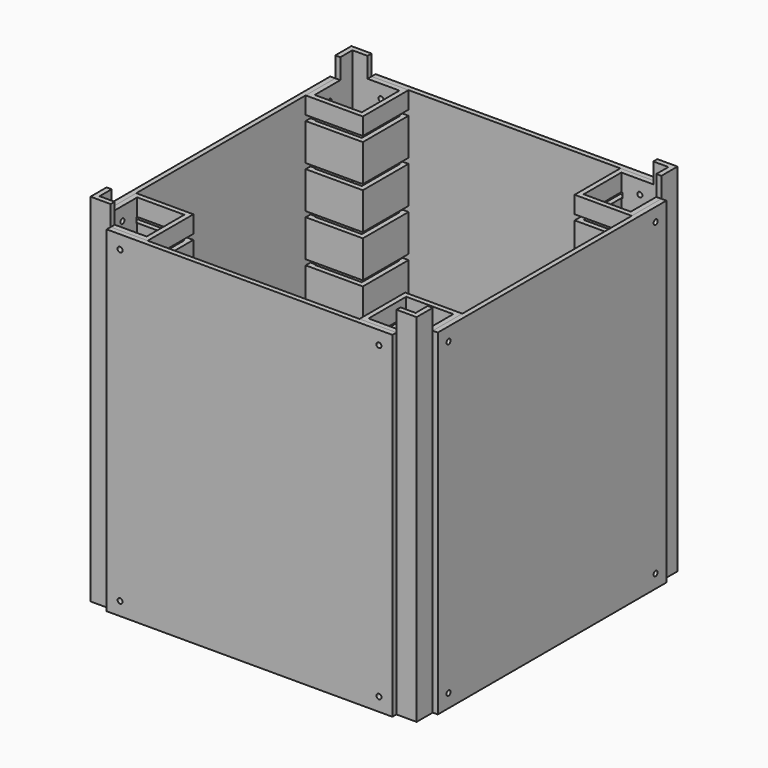
from build123d import *

# Parameters (mm, degrees)
F0_W      = 14
F0_H      = 14
F1_DEPTH  = 100
F2_W      = 85
F2_H      = 1.5
F3_DEPTH  = 100
F2_W_2    = 1.5
F2_H_2    = 85
F5_DEPTH  = 6
F6_R      = 0.75
F7_DEPTH  = 10
F8_R      = 0.75
F9_DEPTH  = 10
F10_R     = 0.75
F11_DEPTH = 10
F12_R     = 0.75
F13_DEPTH = 10
F14_W     = 17
F14_H     = 1.6
F15_DEPTH = 1.8
F16_W     = 17
F16_H     = 1.6
F17_DEPTH = 1.8
F18_W     = 17
F18_H     = 1.6
F19_DEPTH = 1.8
F20_W     = 17
F20_H     = 1.6
F21_DEPTH = 1.8
F22_W     = 17
F22_H     = 1.6
F23_DEPTH = 1.8
F24_W     = 17
F24_H     = 1.6
F25_DEPTH = 1.8
F26_W     = 17
F26_H     = 1.6
F27_DEPTH = 1.8
F28_W     = 17
F28_H     = 1.6
F29_DEPTH = 1.8
F30_W     = 17
F30_H     = 1.6
F31_DEPTH = 1.8
F32_W     = 17
F32_H     = 1.6
F33_DEPTH = 1.8


with BuildPart() as f1:
    # F0 (on Top) → F1 (new body)
    with BuildSketch(Plane.XY):
        Polygon((17, 97), (0, 97), (0, 95.5), (0, 80), (1.5, 80), (15.5, 80), (17, 80), (17, 95.5), align=None)
        with Locations((8.5, 88.5)):
            Rectangle(F0_W, F0_H, mode=Mode.SUBTRACT)
    extrude(amount=-F1_DEPTH)

    # F4 (on face) → F5 (join)
    with BuildSketch(Plane.XY):
        Polygon((6, 97), (0, 97), (0, 91), (1.5, 91), (1.5, 95.5), (6, 95.5), align=None)
    extrude(amount=F5_DEPTH)


with BuildPart() as f1b:
    # F0 (on Top) → F1, piece 2 (new body)
    with BuildSketch(Plane.XY):
        Polygon((97, 97), (80, 97), (80, 95.5), (80, 80), (81.5, 80), (95.5, 80), (97, 80), (97, 95.5), align=None)
        with Locations((88.5, 88.5)):
            Rectangle(F0_W, F0_H, mode=Mode.SUBTRACT)
    extrude(amount=-F1_DEPTH)

    # F4 (on face) → F5, piece 2 (join)
    with BuildSketch(Plane.XY):
        Polygon((97, 97), (91, 97), (91, 95.5), (95.5, 95.5), (95.5, 91), (97, 91), align=None)
    extrude(amount=F5_DEPTH)


with BuildPart() as f1c:
    # F0 (on Top) → F1, piece 3 (new body)
    with BuildSketch(Plane.XY):
        Polygon((95.5, 0), (97, 0), (97, 15.5), (97, 17), (80, 17), (80, 15.5), (80, 0), (81.5, 0), align=None)
        with Locations((88.5, 8.5)):
            Rectangle(F0_W, F0_H, mode=Mode.SUBTRACT)
    extrude(amount=-F1_DEPTH)

    # F4 (on face) → F5, piece 3 (join)
    with BuildSketch(Plane.XY):
        Polygon((97, 0), (97, 6), (95.5, 6), (95.5, 1.5), (91, 1.5), (91, 0), align=None)
    extrude(amount=F5_DEPTH)


with BuildPart() as f1d:
    # F0 (on Top) → F1, piece 4 (new body)
    with BuildSketch(Plane.XY):
        Polygon((17, 15.5), (17, 17), (0, 17), (0, 15.5), (0, 0), (1.5, 0), (15.5, 0), (17, 0), align=None)
        with Locations((8.5, 8.5)):
            Rectangle(F0_W, F0_H, mode=Mode.SUBTRACT)
    extrude(amount=-F1_DEPTH)

    # F4 (on face) → F5, piece 4 (join)
    with BuildSketch(Plane.XY):
        Polygon((1.5, 6), (0, 6), (0, 0), (6, 0), (6, 1.5), (1.5, 1.5), align=None)
    extrude(amount=F5_DEPTH)


with BuildPart() as f3:
    # F2 (on face) → F3 (new body)
    with BuildSketch(Plane.XY):
        with Locations((48.5, -0.75)):
            Rectangle(F2_W, F2_H)
    extrude(amount=-F3_DEPTH)


with BuildPart() as f3b:
    # F2 (on face) → F3, piece 2 (new body)
    with BuildSketch(Plane.XY):
        with Locations((-0.75, 48.5)):
            Rectangle(F2_W_2, F2_H_2)
    extrude(amount=-F3_DEPTH)


with BuildPart() as f3c:
    # F2 (on face) → F3, piece 3 (new body)
    with BuildSketch(Plane.XY):
        Polygon((98.5, 91), (97, 91), (97, 80), (97, 17), (97, 6), (98.5, 6), align=None)
    extrude(amount=-F3_DEPTH)


with BuildPart() as f3d:
    # F2 (on face) → F3, piece 4 (new body)
    with BuildSketch(Plane.XY):
        Polygon((6, 98.5), (6, 97), (80, 97), (91, 97), (91, 98.5), align=None)
    extrude(amount=-F3_DEPTH)


with BuildPart() as f7_tool:
    # F6 (on face) → F7 (new body)
    with BuildSketch(Plane.YZ.offset(98.5)):
        with Locations((10, -4)):
            Circle(F6_R)
        with Locations((87, -4)):
            Circle(F6_R)
        with Locations((87, -96)):
            Circle(F6_R)
        with Locations((10, -96)):
            Circle(F6_R)
    extrude(amount=-F7_DEPTH)


with BuildPart() as f1b_1:
    add(f1b.part)

    # F7: cut by f7_tool
    add(f7_tool.part, mode=Mode.SUBTRACT)


with BuildPart() as f1c_1:
    add(f1c.part)

    # F7: cut by f7_tool
    add(f7_tool.part, mode=Mode.SUBTRACT)


with BuildPart() as f3c_1:
    add(f3c.part)

    # F7: cut by f7_tool
    add(f7_tool.part, mode=Mode.SUBTRACT)


with BuildPart() as f9_tool:
    # F8 (on face) → F9 (new body)
    with BuildSketch(Plane(origin=(0, 98.5, 0), x_dir=(-1, 0, 0), z_dir=(0, 1, 0))):
        with Locations((-87, -4)):
            Circle(F8_R)
        with Locations((-10, -4)):
            Circle(F8_R)
        with Locations((-10, -96)):
            Circle(F8_R)
        with Locations((-87, -96)):
            Circle(F8_R)
    extrude(amount=-F9_DEPTH)


with BuildPart() as f1_1:
    add(f1.part)

    # F9: cut by f9_tool
    add(f9_tool.part, mode=Mode.SUBTRACT)


with BuildPart() as f1b_2:
    add(f1b_1.part)

    # F9: cut by f9_tool
    add(f9_tool.part, mode=Mode.SUBTRACT)

    # F22 (on face) → F23 (cut)
    with BuildSketch(Plane.XZ.offset(-80)):
        with Locations((88.5, -5.91)):
            Rectangle(F22_W, F22_H)
        with Locations((88.5, -18.51)):
            Rectangle(F22_W, F22_H)
        with Locations((88.5, -31.11)):
            Rectangle(F22_W, F22_H)
        with Locations((88.5, -43.71)):
            Rectangle(F22_W, F22_H)
        with Locations((88.5, -56.31)):
            Rectangle(F22_W, F22_H)
        with Locations((88.5, -68.91)):
            Rectangle(F22_W, F22_H)
        with Locations((88.5, -81.51)):
            Rectangle(F22_W, F22_H)
        with Locations((88.5, -94.11)):
            Rectangle(F22_W, F22_H)
    extrude(amount=-F23_DEPTH, mode=Mode.SUBTRACT)

    # F24 (on face) → F25 (cut)
    with BuildSketch(Plane(origin=(80, 0, 0), x_dir=(0, -1, 0), z_dir=(-1, 0, 0))):
        with Locations((-88.5, -5.91)):
            Rectangle(F24_W, F24_H)
        with Locations((-88.5, -18.51)):
            Rectangle(F24_W, F24_H)
        with Locations((-88.5, -31.11)):
            Rectangle(F24_W, F24_H)
        with Locations((-88.5, -43.71)):
            Rectangle(F24_W, F24_H)
        with Locations((-88.5, -56.31)):
            Rectangle(F24_W, F24_H)
        with Locations((-88.5, -68.91)):
            Rectangle(F24_W, F24_H)
        with Locations((-88.5, -81.51)):
            Rectangle(F24_W, F24_H)
        with Locations((-88.5, -94.11)):
            Rectangle(F24_W, F24_H)
    extrude(amount=-F25_DEPTH, mode=Mode.SUBTRACT)


with BuildPart() as f3d_1:
    add(f3d.part)

    # F9: cut by f9_tool
    add(f9_tool.part, mode=Mode.SUBTRACT)


with BuildPart() as f11_tool:
    # F10 (on face) → F11 (new body)
    with BuildSketch(Plane(origin=(-1.5, 0, 0), x_dir=(0, -1, 0), z_dir=(-1, 0, 0))):
        with Locations((-87, -96)):
            Circle(F10_R)
        with Locations((-10, -96)):
            Circle(F10_R)
        with Locations((-10, -4)):
            Circle(F10_R)
        with Locations((-87, -4)):
            Circle(F10_R)
    extrude(amount=-F11_DEPTH)


with BuildPart() as f1_2:
    add(f1_1.part)

    # F11: cut by f11_tool
    add(f11_tool.part, mode=Mode.SUBTRACT)

    # F14 (on face) → F15 (cut)
    with BuildSketch(Plane.XZ.offset(-80)):
        with Locations((8.5, -5.91)):
            Rectangle(F14_W, F14_H)
    extrude(amount=-F15_DEPTH, mode=Mode.SUBTRACT)

    # F16 (on face) → F17 (cut)
    with BuildSketch(Plane.YZ.offset(17)):
        with Locations((88.5, -5.91)):
            Rectangle(F16_W, F16_H)
    extrude(amount=-F17_DEPTH, mode=Mode.SUBTRACT)

    # F18 (on face) → F19 (cut)
    with BuildSketch(Plane.XZ.offset(-80)):
        with Locations((8.5, -94.11)):
            Rectangle(F18_W, F18_H)
        with Locations((8.5, -81.51)):
            Rectangle(F18_W, F18_H)
        with Locations((8.5, -68.91)):
            Rectangle(F18_W, F18_H)
        with Locations((8.5, -56.31)):
            Rectangle(F18_W, F18_H)
        with Locations((8.5, -43.71)):
            Rectangle(F18_W, F18_H)
        with Locations((8.5, -31.11)):
            Rectangle(F18_W, F18_H)
        with Locations((8.5, -18.51)):
            Rectangle(F18_W, F18_H)
    extrude(amount=-F19_DEPTH, mode=Mode.SUBTRACT)

    # F20 (on face) → F21 (cut)
    with BuildSketch(Plane.YZ.offset(17)):
        with Locations((88.5, -18.51)):
            Rectangle(F20_W, F20_H)
        with Locations((88.5, -31.11)):
            Rectangle(F20_W, F20_H)
        with Locations((88.5, -43.71)):
            Rectangle(F20_W, F20_H)
        Polygon((97, -55.51), (81.8, -55.51), (80, -55.51), (80, -57.11), (97, -57.11), align=None)
        with Locations((88.5, -68.91)):
            Rectangle(F20_W, F20_H)
        with Locations((88.5, -81.51)):
            Rectangle(F20_W, F20_H)
        with Locations((88.5, -94.11)):
            Rectangle(F20_W, F20_H)
    extrude(amount=-F21_DEPTH, mode=Mode.SUBTRACT)


with BuildPart() as f1d_1:
    add(f1d.part)

    # F11: cut by f11_tool
    add(f11_tool.part, mode=Mode.SUBTRACT)


with BuildPart() as f3b_1:
    add(f3b.part)

    # F11: cut by f11_tool
    add(f11_tool.part, mode=Mode.SUBTRACT)


with BuildPart() as f13_tool:
    # F12 (on face) → F13 (new body)
    with BuildSketch(Plane.XZ.offset(1.5)):
        with Locations((10, -4)):
            Circle(F12_R)
        with Locations((87, -4)):
            Circle(F12_R)
        with Locations((87, -96)):
            Circle(F12_R)
        with Locations((10, -96)):
            Circle(F12_R)
    extrude(amount=-F13_DEPTH)


with BuildPart() as f1c_2:
    add(f1c_1.part)

    # F13: cut by f13_tool
    add(f13_tool.part, mode=Mode.SUBTRACT)

    # F26 (on face) → F27 (cut)
    with BuildSketch(Plane(origin=(80, 0, 0), x_dir=(0, -1, 0), z_dir=(-1, 0, 0))):
        with Locations((-8.5, -5.91)):
            Rectangle(F26_W, F26_H)
        with Locations((-8.5, -18.51)):
            Rectangle(F26_W, F26_H)
        with Locations((-8.5, -31.11)):
            Rectangle(F26_W, F26_H)
        with Locations((-8.5, -43.71)):
            Rectangle(F26_W, F26_H)
        with Locations((-8.5, -56.31)):
            Rectangle(F26_W, F26_H)
        with Locations((-8.5, -68.91)):
            Rectangle(F26_W, F26_H)
        with Locations((-8.5, -81.51)):
            Rectangle(F26_W, F26_H)
        with Locations((-8.5, -94.11)):
            Rectangle(F26_W, F26_H)
    extrude(amount=-F27_DEPTH, mode=Mode.SUBTRACT)

    # F28 (on face) → F29 (cut)
    with BuildSketch(Plane(origin=(0, 17, 0), x_dir=(-1, 0, 0), z_dir=(0, 1, 0))):
        with Locations((-88.5, -5.91)):
            Rectangle(F28_W, F28_H)
        with Locations((-88.5, -18.51)):
            Rectangle(F28_W, F28_H)
        with Locations((-88.5, -31.11)):
            Rectangle(F28_W, F28_H)
        with Locations((-88.5, -43.71)):
            Rectangle(F28_W, F28_H)
        with Locations((-88.5, -56.31)):
            Rectangle(F28_W, F28_H)
        with Locations((-88.5, -68.91)):
            Rectangle(F28_W, F28_H)
        with Locations((-88.5, -81.51)):
            Rectangle(F28_W, F28_H)
        with Locations((-88.5, -94.11)):
            Rectangle(F28_W, F28_H)
    extrude(amount=-F29_DEPTH, mode=Mode.SUBTRACT)


with BuildPart() as f1d_2:
    add(f1d_1.part)

    # F13: cut by f13_tool
    add(f13_tool.part, mode=Mode.SUBTRACT)

    # F30 (on face) → F31 (cut)
    with BuildSketch(Plane(origin=(0, 17, 0), x_dir=(-1, 0, 0), z_dir=(0, 1, 0))):
        with Locations((-8.5, -5.91)):
            Rectangle(F30_W, F30_H)
        with Locations((-8.5, -18.51)):
            Rectangle(F30_W, F30_H)
        with Locations((-8.5, -31.11)):
            Rectangle(F30_W, F30_H)
        with Locations((-8.5, -43.71)):
            Rectangle(F30_W, F30_H)
        with Locations((-8.5, -56.31)):
            Rectangle(F30_W, F30_H)
        with Locations((-8.5, -68.91)):
            Rectangle(F30_W, F30_H)
        with Locations((-8.5, -81.51)):
            Rectangle(F30_W, F30_H)
        with Locations((-8.5, -94.11)):
            Rectangle(F30_W, F30_H)
    extrude(amount=-F31_DEPTH, mode=Mode.SUBTRACT)

    # F32 (on face) → F33 (cut)
    with BuildSketch(Plane.YZ.offset(17)):
        with Locations((8.5, -5.91)):
            Rectangle(F32_W, F32_H)
        with Locations((8.5, -18.51)):
            Rectangle(F32_W, F32_H)
        with Locations((8.5, -31.11)):
            Rectangle(F32_W, F32_H)
        with Locations((8.5, -43.71)):
            Rectangle(F32_W, F32_H)
        with Locations((8.5, -56.31)):
            Rectangle(F32_W, F32_H)
        with Locations((8.5, -68.91)):
            Rectangle(F32_W, F32_H)
        with Locations((8.5, -81.51)):
            Rectangle(F32_W, F32_H)
        with Locations((8.5, -94.11)):
            Rectangle(F32_W, F32_H)
    extrude(amount=-F33_DEPTH, mode=Mode.SUBTRACT)


with BuildPart() as f3_1:
    add(f3.part)

    # F13: cut by f13_tool
    add(f13_tool.part, mode=Mode.SUBTRACT)


solid = Compound([f3c_1.part, f1b_2.part, f3d_1.part, f1_2.part, f3b_1.part, f1c_2.part, f1d_2.part, f3_1.part])
